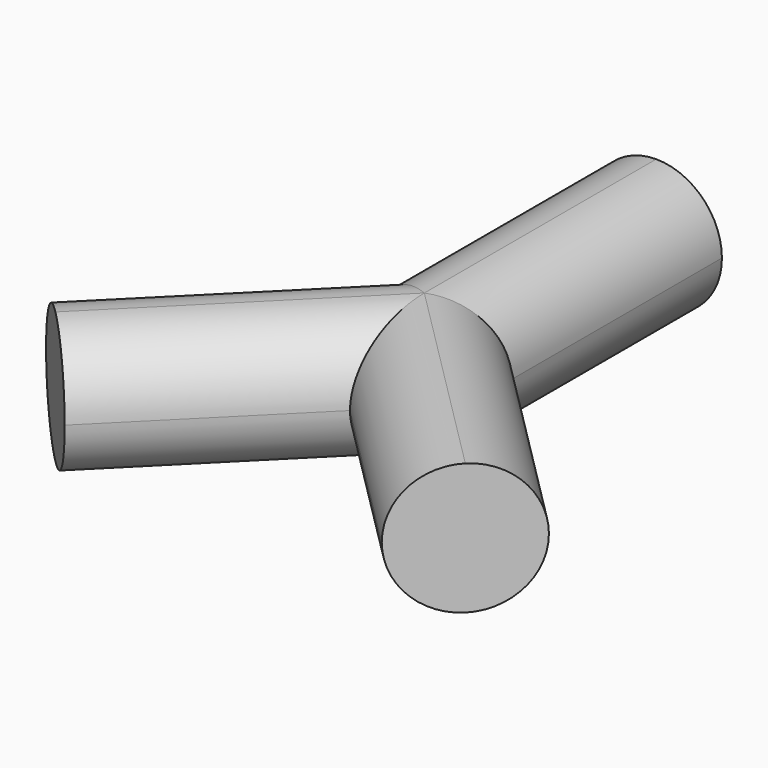
from build123d import *

# Parameters (mm, degrees)
F0_W     = 12.7
F0_H     = 25.4
F1_DEPTH = 6.35
F2_R     = 6.34999


# Not quite as in the source:
# - a fillet or chamfer is up to 0.001 mm smaller than in the source, because OpenCascade refuses the exact size


with BuildPart() as f1:
    # F0 (on Top) → F1 (new body, symmetric)
    with BuildSketch(Plane.XY):
        Polygon((6.35, 0), (-6.35, 0), (-24.3105122421, -17.9605122421), (-15.3302561211, -26.9407683632), (0, -11.6105122421), (15.3302561211, -26.9407683632), (24.3105122421, -17.9605122421), align=None)
        with Locations((0, 12.7)):
            Rectangle(F0_W, F0_H)
    extrude(amount=F1_DEPTH, both=True)

    # F2 (radius 6.35 in the source; OpenCascade refuses exactly that, so slightly less here)
    f2_edges = [f1.edges().sort_by_distance(p)[0] for p in [
        (6.35, 12.7, 6.35),
        (6.35, 12.7, -6.35),
        (-6.35, 12.7, 6.35),
        (-6.35, 12.7, -6.35),
        (15.330256, -8.980256, 6.35),
        (15.330256, -8.980256, -6.35),
        (7.665128, -19.27564, 6.35),
        (7.665128, -19.27564, -6.35),
        (-7.665128, -19.27564, 6.35),
        (-7.665128, -19.27564, -6.35),
        (-15.330256, -8.980256, 6.35),
        (-15.330256, -8.980256, -6.35),
    ]]
    fillet(f2_edges, radius=F2_R)


solid = f1.part
